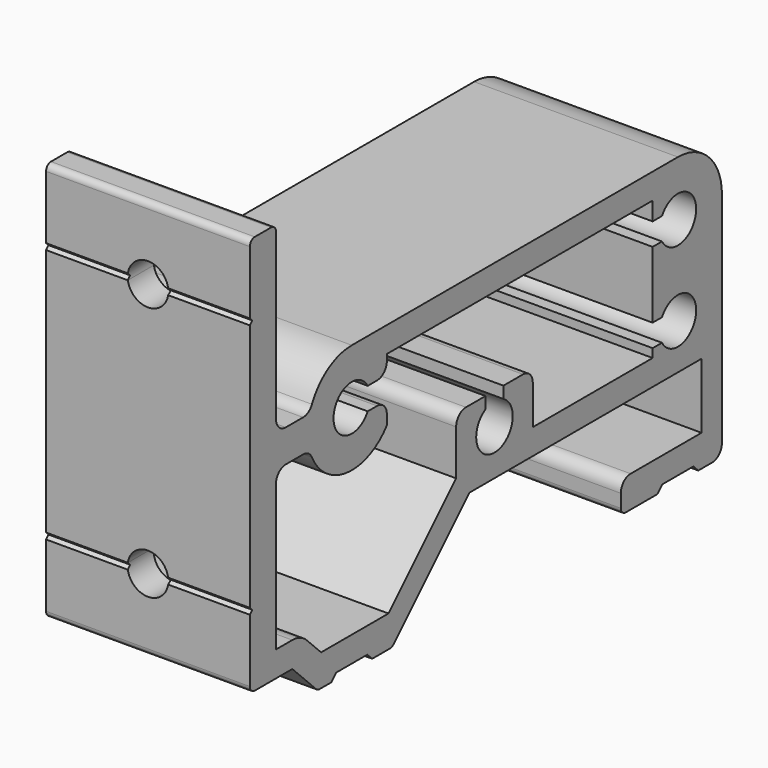
from build123d import *

# Parameters (mm, degrees)
F1_DEPTH = 25.4
F3_DEPTH = 25.4


# Not quite as in the source:
# - ends of sketch curves that miss each other by under 0.0002 mm in the source are joined


with BuildPart() as f1:
    # F0 (on Right) → F1 (new body)
    with BuildSketch(Plane.YZ):
        with BuildLine():
            Line((-36.7665, 26.0985), (-36.7665, 18.2245))
            Line((-36.7665, 18.2245), (-36.3855, 17.8435))
            Line((-36.3855, 17.8435), (-36.7665, 17.4625))
            Line((-36.7665, 17.4625), (-36.7665, -13.5255))
            Line((-36.7665, -13.5255), (-36.3855, -13.9065))
            Line((-36.3855, -13.9065), (-36.7665, -14.2875))
            Line((-36.7665, -14.2875), (-36.7665, -22.1615))
            ThreePointArc((-36.7665, -22.1615), (-36.5433153673, -22.7003153673), (-36.0045, -22.9235))
            Line((-36.0045, -22.9235), (-30.1625, -22.9235))
            Line((-30.1625, -22.9235), (-26.4486898, -26.6373356))
            ThreePointArc((-26.4486898, -26.6373356), (-26.2014589755, -26.8024962038), (-25.9098542, -26.8605))
            Line((-25.9098542, -26.8605), (-24.0665, -26.8605))
            Line((-24.0665, -26.8605), (-23.3045, -26.0985))
            Line((-23.3045, -26.0985), (-18.4785, -26.0985))
            Line((-18.4785, -26.0985), (-17.7165, -26.8605))
            Line((-17.7165, -26.8605), (-14.9389846, -26.8605))
            ThreePointArc((-14.9389846, -26.8605), (-14.6473881211, -26.8024996403), (-14.4001819327, -26.6373280669))
            Line((-14.4001819327, -26.6373280669), (-2.5583642, -14.7955))
            Line((-2.5583642, -14.7955), (33.5915, -14.7955))
            Line((33.5915, -14.7955), (33.5915, -22.9235))
            Line((33.5915, -22.9235), (22.5425, -22.9235))
            ThreePointArc((22.5425, -22.9235), (21.4648692655, -23.3698692655), (21.0185, -24.4475))
            Line((21.0185, -24.4475), (21.0185, -26.0985))
            ThreePointArc((21.0185, -26.0985), (21.2416846327, -26.6373153673), (21.7805, -26.8605))
            Line((21.7805, -26.8605), (26.7335, -26.8605))
            Line((26.7335, -26.8605), (27.4955, -26.0985))
            Line((27.4955, -26.0985), (32.3215, -26.0985))
            Line((32.3215, -26.0985), (33.0835, -26.8605))
            Line((33.0835, -26.8605), (35.2425, -26.8605))
            ThreePointArc((35.2425, -26.8605), (36.3201307345, -26.4141307345), (36.7665, -25.3365))
            Line((36.7665, -25.3365), (36.7665, 1.9685))
            ThreePointArc((36.7665, 1.9685), (34.7578383054, 6.8178383054), (29.9085, 8.8265))
            Line((29.9085, 8.8265), (-20.8915, 8.8265))
            ThreePointArc((-20.8915, 8.8265), (-24.5711182212, 7.7557768852), (-27.1017564824, 4.8779464117))
            ThreePointArc((-27.1017564824, 4.8779464117), (-27.6641193484, 4.2384353631), (-28.4818074, 4.0005))
            Line((-28.4818074, 4.0005), (-31.1785, 4.0005))
            ThreePointArc((-31.1785, 4.0005), (-32.2561307345, 4.4468692655), (-32.7025, 5.5245))
            Line((-32.7025, 5.5245), (-32.7025, 26.0985))
            ThreePointArc((-32.7025, 26.0985), (-32.9256846327, 26.6373153673), (-33.4645, 26.8605))
            Line((-33.4645, 26.8605), (-36.0045, 26.8605))
            ThreePointArc((-36.0045, 26.8605), (-36.5433153673, 26.6373153673), (-36.7665, 26.0985))
        make_face()
        with BuildLine():
            Line((-18.4133236, 3.3655), (-16.9545, 3.3655))
            ThreePointArc((-16.9545, 3.3655), (-15.8768692655, 3.8118692655), (-15.4305, 4.8895))
            Line((-15.4305, 4.8895), (-15.4305, 5.6515))
            Line((-15.4305, 5.6515), (25.9715, 5.6515))
            Line((25.9715, 5.6515), (25.9715, 3.3655))
            Line((25.9715, 3.3655), (27.430349, 3.3655))
            ThreePointArc((27.430349, 3.3655), (32.7533, 1.9685), (27.4303420089, 0.5714960589))
            Line((27.4303420089, 0.5714960589), (25.9715, 0.5715))
            Line((25.9715, 0.5715), (25.9715, -7.747))
            Line((25.9715, -7.747), (27.430349, -7.747))
            ThreePointArc((27.430349, -7.747), (32.7533, -9.144), (27.4303420089, -10.5410039411))
            Line((27.4303420089, -10.5410039411), (25.9715, -10.541))
            Line((25.9715, -10.541), (25.9715, -11.6205))
            Line((25.9715, -11.6205), (7.3025, -11.6205))
            Line((7.3025, -11.6205), (7.3025, -6.731))
            ThreePointArc((7.3025, -6.731), (6.8561307345, -5.6533692655), (5.7785, -5.207))
            Line((5.7785, -5.207), (2.7305, -5.207))
            Line((2.7305, -5.207), (2.7305, -6.665849))
            ThreePointArc((2.7305, -6.665849), (1.3335, -11.9888), (-0.0635039411, -6.6658420089))
            Line((-0.0635039411, -6.6658420089), (-0.0635, -5.207))
            Line((-0.0635, -5.207), (-3.1115, -5.207))
            ThreePointArc((-3.1115, -5.207), (-4.1891307345, -5.6533692655), (-4.6355, -6.731))
            Line((-4.6355, -6.731), (-4.6355, -12.3825))
            Line((-4.6355, -12.3825), (-15.1765, -22.9235))
            Line((-15.1765, -22.9235), (-25.6723642, -22.9235))
            Line((-25.6723642, -22.9235), (-27.9174194, -20.6784448))
            ThreePointArc((-27.9174194, -20.6784448), (-28.9474718056, -19.9901859209), (-30.1625, -19.7485))
            Line((-30.1625, -19.7485), (-32.7025, -19.7485))
            Line((-32.7025, -19.7485), (-32.7025, -1.5875))
            ThreePointArc((-32.7025, -1.5875), (-32.2561307345, -0.5098692655), (-31.1785, -0.0635))
            Line((-31.1785, -0.0635), (-28.4818074, -0.0635))
            ThreePointArc((-28.4818074, -0.0635), (-27.6641096434, -0.3014415336), (-27.1017455591, -0.9409666943))
            ThreePointArc((-27.1017455591, -0.9409666943), (-21.615457962, -4.8511809947), (-15.4305020835, -2.1799534173))
            Line((-15.4305020835, -2.1799534173), (-15.4305, -0.9525))
            ThreePointArc((-15.4305, -0.9525), (-15.8768692655, 0.1251307345), (-16.9545, 0.5715))
            Line((-16.9545, 0.5715), (-18.4133236, 0.5715))
            ThreePointArc((-18.4133236, 0.5715), (-23.7363, 1.9685), (-18.4133236, 3.3655))
        make_face(mode=Mode.SUBTRACT)
    extrude(amount=F1_DEPTH)

    # F2 (on face) → F3 (cut)
    with BuildSketch(Plane.XZ.offset(36.7665)):
        with BuildLine():
            ThreePointArc((10.1889011104, 17.4625), (12.8915839509, 15.311811972), (15.24, 17.8445763886))
            ThreePointArc((15.24, 17.8445763886), (12.5084160491, 20.3773408052), (10.1889011104, 17.4625))
        make_face()
        with BuildLine():
            ThreePointArc((10.1887375685, -13.5255), (12.5089588736, -16.4393054185), (15.24, -13.9065))
            ThreePointArc((15.24, -13.9065), (12.8910411264, -11.3736945815), (10.1887375685, -13.5255))
        make_face()
    extrude(amount=-F3_DEPTH, mode=Mode.SUBTRACT)


solid = f1.part
